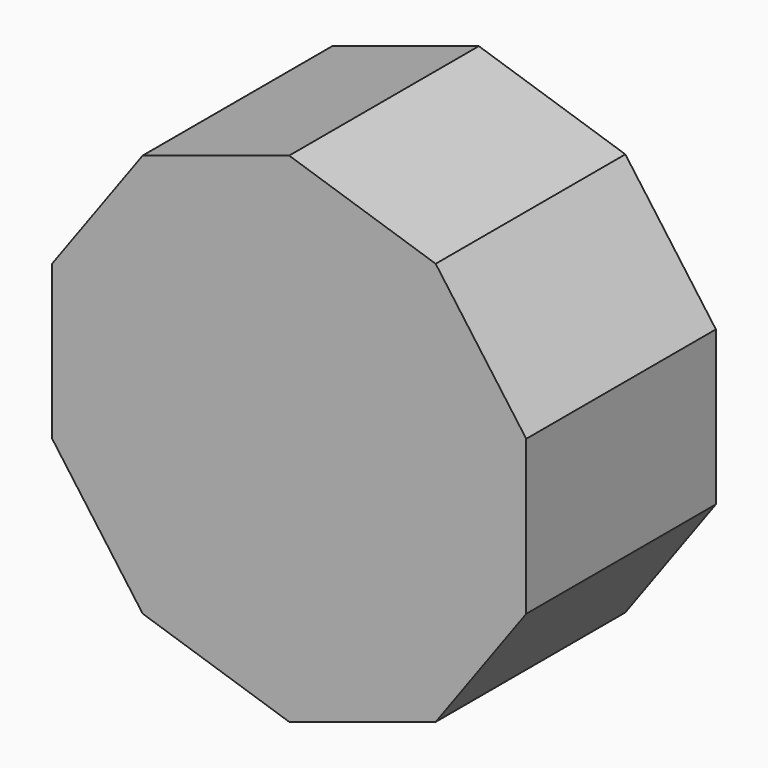
from build123d import *

# Parameters (mm, degrees)
F1_DEPTH = 6.35


# Not quite as in the source:
# - the program builds the solid bodies; features that only make, move or delete a surface that nothing else refers to are left out


with BuildPart() as f1:
    # F0 (on Front) → F1 (new body)
    with BuildSketch(Plane.XZ):
        Polygon((6.35, -2.0632400711), (6.35, 2.0632400711), (3.9245158286, 5.401632633), (0, 6.6767851239), (-3.9245158286, 5.401632633), (-6.35, 2.0632400711), (-6.35, -2.0632400711), (-3.9245158286, -5.401632633), (0, -6.6767851239), (3.9245158286, -5.401632633), align=None)
    extrude(amount=F1_DEPTH)


solid = f1.part
